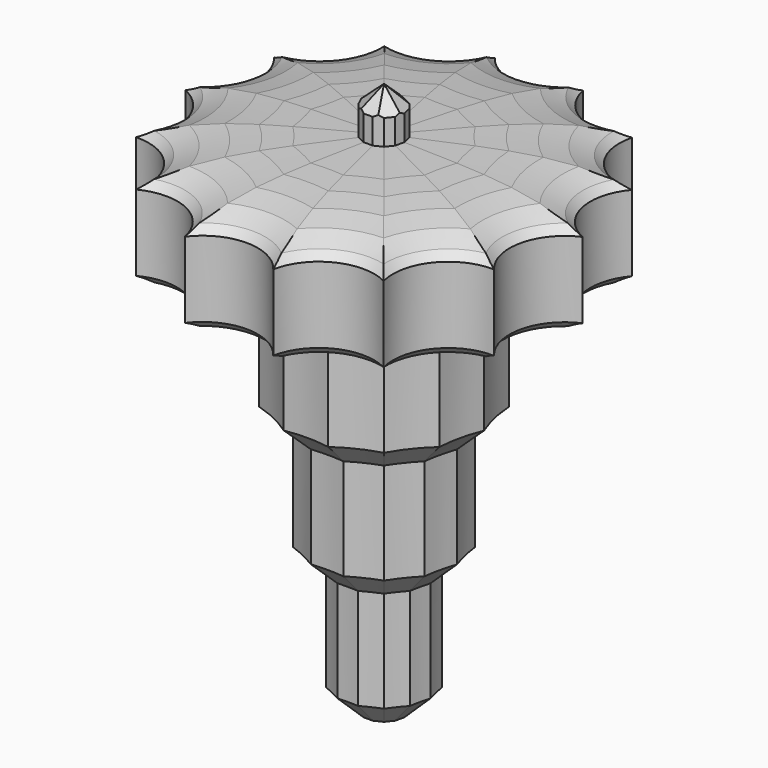
from build123d import *

# Parameters (mm, degrees)
F1_DEPTH      = 25
F2_T2_ANGLE   = 240.9081549798
F2_T4_ANGLE   = 240.9081549798
F2_T6_ANGLE   = 240.9081549797
F2_T8_ANGLE   = 240.9081549798
F2_T10_ANGLE  = 240.9081549798
F2_T12_ANGLE  = 240.9081549798
F2_T14_ANGLE  = 240.9081549798
F2_T16_ANGLE  = 240.9081549798
F2_T18_ANGLE  = 240.9081549798
F2_T20_ANGLE  = 240.9081549798
F2_T22_ANGLE  = 240.9081549798
F2_T24_ANGLE  = 240.9081549797
F2_T26_ANGLE  = 240.9081549798
F2_T28_ANGLE  = 240.9081549798
F3_SIZE       = 5
F4_SIZE       = 5
F5_SIZE       = 5
F6_T2_ANGLE   = 60.0762821523
F6_T4_ANGLE   = 60.0762821523
F6_T6_ANGLE   = 60.0762821523
F6_T8_ANGLE   = 60.0762821523
F6_T10_ANGLE  = 60.0762821523
F6_T12_ANGLE  = 60.0762821523
F6_T14_ANGLE  = 60.0762821523
F6_T16_ANGLE  = 60.0762821523
F6_T18_ANGLE  = 60.0762821523
F6_T20_ANGLE  = 60.0762821523
F6_T22_ANGLE  = 60.0762821523
F6_T24_ANGLE  = 60.0762821523
F6_T26_ANGLE  = 60.0762821523
F6_T28_ANGLE  = 60.0762821523
F7_T2_ANGLE   = 47.9835286681
F7_T4_ANGLE   = 47.9835286681
F7_T6_ANGLE   = 47.9835286681
F7_T8_ANGLE   = 47.9835286681
F7_T10_ANGLE  = 47.9835286681
F7_T12_ANGLE  = 47.9835286681
F7_T14_ANGLE  = 47.9835286681
F7_T16_ANGLE  = 47.9835286681
F7_T18_ANGLE  = 47.9835286681
F7_T20_ANGLE  = 47.9835286681
F7_T22_ANGLE  = 47.9835286681
F7_T24_ANGLE  = 47.9835286681
F7_T26_ANGLE  = 47.9835286681
F7_T28_ANGLE  = 47.9835286681
F8_T2_ANGLE   = 240.9081549798
F8_T4_ANGLE   = 240.9081549798
F8_T6_ANGLE   = 240.9081549798
F8_T8_ANGLE   = 240.9081549798
F8_T10_ANGLE  = 240.9081549798
F8_T12_ANGLE  = 240.9081549798
F8_T14_ANGLE  = 240.9081549797
F8_T16_ANGLE  = 240.9081549798
F8_T18_ANGLE  = 240.9081549797
F8_T20_ANGLE  = 240.9081549798
F8_T22_ANGLE  = 240.9081549798
F8_T24_ANGLE  = 240.9081549798
F8_T26_ANGLE  = 240.9081549798
F8_T28_ANGLE  = 240.9081549798
F9_SIZE       = 5
F10_SIZE      = 5
F11_DEPTH     = 25
F12_DEPTH     = 10
F13_T2_ANGLE  = 76.3607936653
F13_T4_ANGLE  = 76.3607936653
F13_T6_ANGLE  = 76.3607936653
F13_T8_ANGLE  = 76.3607936653
F13_T10_ANGLE = 76.3607936653
F13_T12_ANGLE = 76.3607936653
F13_T14_ANGLE = 76.3607936653
F13_T16_ANGLE = 76.3607936653
F13_T18_ANGLE = 76.3607936653
F13_T20_ANGLE = 76.3607936653
F13_T22_ANGLE = 76.3607936653
F13_T24_ANGLE = 76.3607936653
F13_T26_ANGLE = 76.3607936653
F13_T28_ANGLE = 76.3607936653
F13_T30_ANGLE = 38.4969644014
F13_T32_ANGLE = 38.4969644014
F13_T34_ANGLE = 38.4969644014
F13_T36_ANGLE = 38.4969644014
F13_T38_ANGLE = 38.4969644015
F13_T40_ANGLE = 38.4969644015
F13_T42_ANGLE = 38.4969644015
F15_DEPTH     = 25
F16_SIZE      = 5
F17_DEPTH     = 25
F18_SIZE      = 5


# Not quite as in the source:
# - a fillet or chamfer that OpenCascade refuses, or shapes differently, is made with other operations: its cross-section is extruded or revolved along the edge and cut away or added
# - two fillets or chamfers of one size are made in one step


with BuildPart() as f1:
    # F0 (on Top) → F1 (new body)
    with BuildSketch(Plane.XY):
        with BuildLine():
            ThreePointArc((24.463741661, 30.6765617538), (14.7080431141, 30.541566228), (8.731008312, 38.2530468191))
            ThreePointArc((8.731008312, 38.2530468191), (0, 33.8985810899), (-8.731008312, 38.2530468191))
            ThreePointArc((-8.731008312, 38.2530468191), (-14.7080431141, 30.541566228), (-24.463741661, 30.6765617538))
            ThreePointArc((-24.463741661, 30.6765617538), (-24.2050150864, 29.3243775762), (-24.1183144167, 27.9503963229))
            ThreePointArc((-24.1183144167, 27.9503963229), (-27.4274265196, 20.1152547902), (-35.351130946, 17.0242074097))
            ThreePointArc((-35.351130946, 17.0242074097), (-33.4389393825, 13.7278579439), (-32.7746255912, 9.9753809536))
            ThreePointArc((-32.7746255912, 9.9753809536), (-34.53133563, 4.0325730915), (-39.236795194, 0))
            ThreePointArc((-39.236795194, 0), (-34.53133563, -4.0325730915), (-32.7746255912, -9.9753809536))
            ThreePointArc((-32.7746255912, -9.9753809536), (-33.4389393825, -13.7278579439), (-35.351130946, -17.0242074097))
            ThreePointArc((-35.351130946, -17.0242074097), (-27.4274265195, -20.1152547902), (-24.1183144167, -27.9503963229))
            ThreePointArc((-24.1183144167, -27.9503963229), (-24.2050150864, -29.3243775762), (-24.463741661, -30.6765617538))
            ThreePointArc((-24.463741661, -30.6765617538), (-14.7080431141, -30.541566228), (-8.731008312, -38.2530468191))
            ThreePointArc((-8.731008312, -38.2530468191), (0, -33.8985810899), (8.731008312, -38.2530468191))
            ThreePointArc((8.731008312, -38.2530468191), (14.7080431141, -30.541566228), (24.463741661, -30.6765617538))
            ThreePointArc((24.463741661, -30.6765617538), (26.5029779071, -21.135419607), (35.351130946, -17.0242074097))
            ThreePointArc((35.351130946, -17.0242074097), (33.0486728879, -7.5431439239), (39.236795194, 0))
            ThreePointArc((39.236795194, 0), (33.0486728879, 7.5431439239), (35.351130946, 17.0242074097))
            ThreePointArc((35.351130946, 17.0242074097), (26.5029779071, 21.135419607), (24.463741661, 30.6765617538))
        make_face()
    extrude(amount=F1_DEPTH)

    # F2: chamfer of 5 on 14 edges, made by hand

    # F2_s1 → F2_t2 (revolve, cut)
    with BuildSketch(Plane(origin=(-13.8327660938, 36.0835914665, 0), x_dir=(0, 0, 1), z_dir=(-0.357952317, 0.9337398668, 0))):
        Polygon((25, -38.6518225177), (20, -33.6518225177), (25, -33.6518225177), align=None)
    revolve(axis=Axis((-35.0486884109, 27.9503963229, 25), (0, 0, 1)), revolution_arc=F2_T2_ANGLE, mode=Mode.SUBTRACT)

    # F2_s3 → F2_t4 (revolve, cut)
    with BuildSketch(Plane(origin=(-32.100820462, 21.5153042411, 0), x_dir=(0, 0, 1), z_dir=(-0.8306771749, 0.5567543723, 0))):
        Polygon((25, 38.6518225177), (20, 33.6518225177), (25, 33.6518225177), align=None)
    revolve(axis=Axis((-19.4505546526, 40.3894929114, 25), (0, 0, -1)), revolution_arc=F2_T4_ANGLE, mode=Mode.SUBTRACT)

    # F2_s5 → F2_t6 (revolve, cut)
    with BuildSketch(Plane(origin=(-19.586699218, 33.3126433155, 0), x_dir=(0, 0, 1), z_dir=(-0.5068476051, 0.8620356751, 0))):
        Polygon((25, 38.6518225177), (20, 33.6518225177), (25, 33.6518225177), align=None)
    revolve(axis=Axis((0, 44.8289550841, 25), (0, 0, -1)), revolution_arc=F2_T6_ANGLE, mode=Mode.SUBTRACT)

    # F2_s7 → F2_t8 (revolve, cut)
    with BuildSketch(Plane(origin=(-3.1931919788, 38.5120048285, 0), x_dir=(0, 0, 1), z_dir=(-0.082630651, 0.9965802404, 0))):
        Polygon((25, 38.6518225177), (20, 33.6518225177), (25, 33.6518225177), align=None)
    revolve(axis=Axis((19.4505546526, 40.3894929114, 25), (0, 0, -1)), revolution_arc=F2_T8_ANGLE, mode=Mode.SUBTRACT)

    # F2_s9 → F2_t10 (revolve, cut)
    with BuildSketch(Plane(origin=(13.8327660938, 36.0835914665, 0), x_dir=(0, 0, 1), z_dir=(0.357952317, 0.9337398668, 0))):
        Polygon((25, 38.6518225177), (20, 33.6518225177), (25, 33.6518225177), align=None)
    revolve(axis=Axis((35.0486884109, 27.9503963229, 25), (0, 0, -1)), revolution_arc=F2_T10_ANGLE, mode=Mode.SUBTRACT)

    # F2_s11 → F2_t12 (revolve, cut)
    with BuildSketch(Plane(origin=(28.1189751937, 26.5083802783, 0), x_dir=(0, 0, 1), z_dir=(0.7276384385, 0.685960861, 0))):
        Polygon((25, 38.6518225177), (20, 33.6518225177), (25, 33.6518225177), align=None)
    revolve(axis=Axis((43.7049995854, 9.9753809536, 25), (0, 0, -1)), revolution_arc=F2_T12_ANGLE, mode=Mode.SUBTRACT)

    # F2_s13 → F2_t14 (revolve, cut)
    with BuildSketch(Plane(origin=(36.8358764, 11.682859272, 0), x_dir=(0, 0, 1), z_dir=(0.9532068434, 0.3023188939, 0))):
        Polygon((25, 38.6518225177), (20, 33.6518225177), (25, 33.6518225177), align=None)
    revolve(axis=Axis((43.7049995854, -9.9753809536, 25), (0, 0, -1)), revolution_arc=F2_T14_ANGLE, mode=Mode.SUBTRACT)

    # F2_s15 → F2_t16 (revolve, cut)
    with BuildSketch(Plane(origin=(38.2569805228, -5.4565952939, 0), x_dir=(0, 0, 1), z_dir=(0.9899809427, -0.1412010378, 0))):
        Polygon((20, 33.6518225177), (25, 38.6518225177), (25, 33.6518225177), align=None)
    revolve(axis=Axis((35.0486884109, -27.9503963229, 25), (0, 0, -1)), revolution_arc=F2_T16_ANGLE, mode=Mode.SUBTRACT)

    # F2_s17 → F2_t18 (revolve, cut)
    with BuildSketch(Plane(origin=(32.100820462, -21.5153042411, 0), x_dir=(0, 0, 1), z_dir=(0.8306771749, -0.5567543723, 0))):
        Polygon((25, 38.6518225177), (20, 33.6518225177), (25, 33.6518225177), align=None)
    revolve(axis=Axis((19.4505546526, -40.3894929114, 25), (0, 0, -1)), revolution_arc=F2_T18_ANGLE, mode=Mode.SUBTRACT)

    # F2_s19 → F2_t20 (revolve, cut)
    with BuildSketch(Plane(origin=(19.586699218, -33.3126433155, 0), x_dir=(0, 0, 1), z_dir=(0.5068476051, -0.8620356751, 0))):
        Polygon((25, 38.6518225177), (20, 33.6518225177), (25, 33.6518225177), align=None)
    revolve(axis=Axis((0, -44.8289550841, 25), (0, 0, -1)), revolution_arc=F2_T20_ANGLE, mode=Mode.SUBTRACT)

    # F2_s21 → F2_t22 (revolve, cut)
    with BuildSketch(Plane(origin=(3.1931919788, -38.5120048285, 0), x_dir=(0, 0, 1), z_dir=(0.082630651, -0.9965802404, 0))):
        Polygon((25, 38.6518225177), (20, 33.6518225177), (25, 33.6518225177), align=None)
    revolve(axis=Axis((-19.4505546526, -40.3894929114, 25), (0, 0, -1)), revolution_arc=F2_T22_ANGLE, mode=Mode.SUBTRACT)

    # F2_s23 → F2_t24 (revolve, cut)
    with BuildSketch(Plane(origin=(-38.2569805228, -5.4565952939, 0), x_dir=(0, 0, 1), z_dir=(-0.9899809427, -0.1412010378, 0))):
        Polygon((25, -38.6518225177), (20, -33.6518225177), (25, -33.6518225177), align=None)
    revolve(axis=Axis((-35.0486884109, -27.9503963229, 25), (0, 0, 1)), revolution_arc=F2_T24_ANGLE, mode=Mode.SUBTRACT)

    # F2_s25 → F2_t26 (revolve, cut)
    with BuildSketch(Plane(origin=(-36.8358764, 11.682859272, 0), x_dir=(0, 0, 1), z_dir=(-0.9532068434, 0.3023188939, 0))):
        Polygon((25, -38.6518225177), (20, -33.6518225177), (25, -33.6518225177), align=None)
    revolve(axis=Axis((-43.7049995854, -9.9753809536, 25), (0, 0, 1)), revolution_arc=F2_T26_ANGLE, mode=Mode.SUBTRACT)

    # F2_s27 → F2_t28 (revolve, cut)
    with BuildSketch(Plane(origin=(-28.1189751937, 26.5083802783, 0), x_dir=(0, 0, 1), z_dir=(-0.7276384385, 0.685960861, 0))):
        Polygon((25, -38.6518225177), (20, -33.6518225177), (25, -33.6518225177), align=None)
    revolve(axis=Axis((-43.7049995854, 9.9753809536, 25), (0, 0, 1)), revolution_arc=F2_T28_ANGLE, mode=Mode.SUBTRACT)

    # F3
    f3_edges = [f1.edges().sort_by_distance(p)[0] for p in [
        (-22.59382, 18.017971, 25),
        (-12.538624, 26.036722, 25),
        (0, 28.898581, 25),
        (12.538624, 26.036722, 25),
        (22.59382, 18.017971, 25),
        (28.174033, 6.430539, 25),
        (28.174033, -6.430539, 25),
        (22.59382, -18.017971, 25),
        (12.538624, -26.036722, 25),
        (0, -28.898581, 25),
        (-12.538624, -26.036722, 25),
        (-22.59382, -18.017971, 25),
        (-28.174033, -6.430539, 25),
        (-28.174033, 6.430539, 25),
    ]]
    chamfer(f3_edges, length=F3_SIZE)

    # F4
    f4_edges = [f1.edges().sort_by_distance(p)[0] for p in [
        (-18.684663, 14.900522, 25),
        (-10.369206, 21.531878, 25),
        (0, 23.898581, 25),
        (10.369206, 21.531878, 25),
        (18.684663, 14.900522, 25),
        (23.299394, 5.317935, 25),
        (23.299394, -5.317935, 25),
        (18.684663, -14.900522, 25),
        (10.369206, -21.531878, 25),
        (0, -23.898581, 25),
        (-10.369206, -21.531878, 25),
        (-18.684663, -14.900522, 25),
        (-23.299394, -5.317935, 25),
        (-23.299394, 5.317935, 25),
    ]]
    chamfer(f4_edges, length=F4_SIZE)

    # F5
    f5_edges = [f1.edges().sort_by_distance(p)[0] for p in [
        (-14.775506, 11.783073, 25),
        (-18.424754, 4.20533, 25),
        (-18.424754, -4.20533, 25),
        (-14.775506, -11.783073, 25),
        (-8.199787, -17.027033, 25),
        (0, -18.898581, 25),
        (8.199787, -17.027033, 25),
        (14.775506, -11.783073, 25),
        (-8.199787, 17.027033, 25),
        (0, 18.898581, 25),
        (8.199787, 17.027033, 25),
        (14.775506, 11.783073, 25),
        (18.424754, 4.20533, 25),
        (18.424754, -4.20533, 25),
    ]]
    chamfer(f5_edges, length=F5_SIZE)

    # F6: chamfer of 5 on 14 edges, made by hand

    # F6_s1 → F6_t2 (revolve, cut)
    with BuildSketch(Plane(origin=(-20.8945545214, -8.184460814, 0), x_dir=(0, 0, 1), z_dir=(-0.9311167453, -0.3647212726, 0))):
        Polygon((25, 2.8777102985), (24.5099142984, 12.8536339319), (25, 7.8777102985), align=None)
    revolve(axis=Axis((-35.0486884109, 27.9503963229, 25), (0, 0, 1)), revolution_arc=F6_T2_ANGLE, mode=Mode.SUBTRACT)

    # F6_s3 → F6_t4 (revolve, cut)
    with BuildSketch(Plane(origin=(-15.2742386719, -16.4397518369, 0), x_dir=(0, 0, 1), z_dir=(-0.6806605704, -0.732598927, 0))):
        Polygon((25, 2.8777102985), (24.5099142984, 12.8536339319), (25, 7.8777102985), align=None)
    revolve(axis=Axis((-43.7049995854, 9.9753809536, 25), (0, 0, 1)), revolution_arc=F6_T4_ANGLE, mode=Mode.SUBTRACT)

    # F6_s5 → F6_t6 (revolve, cut)
    with BuildSketch(Plane(origin=(12.6287350804, 18.5494705513, 0), x_dir=(0, 0, 1), z_dir=(0.5627699166, 0.8266135863, 0))):
        Polygon((25, -2.8777102985), (24.5099142984, -12.8536339319), (25, -7.8777102985), align=None)
    revolve(axis=Axis((-19.4505546526, 40.3894929114, 25), (0, 0, -1)), revolution_arc=F6_T6_ANGLE, mode=Mode.SUBTRACT)

    # F6_s7 → F6_t8 (revolve, cut)
    with BuildSketch(Plane(origin=(-6.6286725271, -21.4389483882, 0), x_dir=(0, 0, 1), z_dir=(-0.2953912218, -0.9553763793, 0))):
        Polygon((25, 2.8777102985), (24.5099142984, 12.8536339319), (25, 7.8777102985), align=None)
    revolve(axis=Axis((-43.7049995854, -9.9753809536, 25), (0, 0, 1)), revolution_arc=F6_T8_ANGLE, mode=Mode.SUBTRACT)

    # F6_s9 → F6_t10 (revolve, cut)
    with BuildSketch(Plane(origin=(19.4264107899, 11.2330926858, 0), x_dir=(0, 0, 1), z_dir=(0.8656923682, 0.5005763913, 0))):
        Polygon((25, -2.8777102985), (24.5099142984, -12.8536339318), (25, -7.8777102985), align=None)
    revolve(axis=Axis((0, 44.8289550841, 25), (0, 0, -1)), revolution_arc=F6_T10_ANGLE, mode=Mode.SUBTRACT)

    # F6_s11 → F6_t12 (revolve, cut)
    with BuildSketch(Plane(origin=(3.329783507, -22.1918982798, 0), x_dir=(0, 0, 1), z_dir=(0.148383981, -0.9889298227, 0))):
        Polygon((25, 2.8777102985), (24.5099142984, 12.8536339318), (25, 7.8777102985), align=None)
    revolve(axis=Axis((-35.0486884109, -27.9503963229, 25), (0, 0, 1)), revolution_arc=F6_T12_ANGLE, mode=Mode.SUBTRACT)

    # F6_s13 → F6_t14 (revolve, cut)
    with BuildSketch(Plane(origin=(22.3764475931, 1.691863049, 0), x_dir=(0, 0, 1), z_dir=(0.9971538294, 0.0753939029, 0))):
        Polygon((25, -2.8777102985), (24.5099142984, -12.8536339319), (25, -7.8777102985), align=None)
    revolve(axis=Axis((19.4505546526, 40.3894929114, 25), (0, 0, -1)), revolution_arc=F6_T14_ANGLE, mode=Mode.SUBTRACT)

    # F6_s15 → F6_t16 (revolve, cut)
    with BuildSketch(Plane(origin=(-22.3764475931, -1.691863049, 0), x_dir=(0, 0, 1), z_dir=(-0.9971538294, -0.0753939029, 0))):
        Polygon((25, -2.8777102985), (24.5099142984, -12.8536339319), (25, -7.8777102985), align=None)
    revolve(axis=Axis((-19.4505546526, -40.3894929114, 25), (0, 0, -1)), revolution_arc=F6_T16_ANGLE, mode=Mode.SUBTRACT)

    # F6_s17 → F6_t18 (revolve, cut)
    with BuildSketch(Plane(origin=(20.8945545214, -8.184460814, 0), x_dir=(0, 0, 1), z_dir=(0.9311167453, -0.3647212726, 0))):
        Polygon((25, -2.8777102985), (24.5099142984, -12.8536339319), (25, -7.8777102985), align=None)
    revolve(axis=Axis((35.0486884109, 27.9503963229, 25), (0, 0, -1)), revolution_arc=F6_T18_ANGLE, mode=Mode.SUBTRACT)

    # F6_s19 → F6_t20 (revolve, cut)
    with BuildSketch(Plane(origin=(-19.4264107899, -11.2330926858, 0), x_dir=(0, 0, 1), z_dir=(-0.8656923682, -0.5005763913, 0))):
        Polygon((25, -2.8777102985), (24.5099142984, -12.8536339318), (25, -7.8777102985), align=None)
    revolve(axis=Axis((0, -44.8289550841, 25), (0, 0, -1)), revolution_arc=F6_T20_ANGLE, mode=Mode.SUBTRACT)

    # F6_s21 → F6_t22 (revolve, cut)
    with BuildSketch(Plane(origin=(15.2742386718, -16.4397518369, 0), x_dir=(0, 0, 1), z_dir=(0.6806605704, -0.732598927, 0))):
        Polygon((25, -2.8777102985), (24.5099142984, -12.8536339319), (25, -7.8777102985), align=None)
    revolve(axis=Axis((43.7049995854, 9.9753809536, 25), (0, 0, -1)), revolution_arc=F6_T22_ANGLE, mode=Mode.SUBTRACT)

    # F6_s23 → F6_t24 (revolve, cut)
    with BuildSketch(Plane(origin=(-12.6287350804, -18.5494705513, 0), x_dir=(0, 0, 1), z_dir=(-0.5627699166, -0.8266135863, 0))):
        Polygon((24.5099142984, -12.8536339319), (25, -2.8777102985), (25, -7.8777102985), align=None)
    revolve(axis=Axis((19.4505546526, -40.3894929114, 25), (0, 0, -1)), revolution_arc=F6_T24_ANGLE, mode=Mode.SUBTRACT)

    # F6_s25 → F6_t26 (revolve, cut)
    with BuildSketch(Plane(origin=(6.6286725271, -21.4389483882, 0), x_dir=(0, 0, 1), z_dir=(0.2953912218, -0.9553763793, 0))):
        Polygon((25, -2.8777102985), (24.5099142984, -12.8536339318), (25, -7.8777102985), align=None)
    revolve(axis=Axis((43.7049995854, -9.9753809536, 25), (0, 0, -1)), revolution_arc=F6_T26_ANGLE, mode=Mode.SUBTRACT)

    # F6_s27 → F6_t28 (revolve, cut)
    with BuildSketch(Plane(origin=(-3.329783507, -22.1918982798, 0), x_dir=(0, 0, 1), z_dir=(-0.148383981, -0.9889298227, 0))):
        Polygon((24.5099142984, -12.8536339319), (25, -2.8777102985), (25, -7.8777102985), align=None)
    revolve(axis=Axis((35.0486884109, -27.9503963229, 25), (0, 0, -1)), revolution_arc=F6_T28_ANGLE, mode=Mode.SUBTRACT)

    # F7: chamfer of 5 on 14 edges, made by hand

    # F7_s1 → F7_t2 (revolve, cut)
    with BuildSketch(Plane(origin=(-16.1774332378, -8.3987740904, 0), x_dir=(0, 0, 1), z_dir=(-0.8875195673, -0.4607700268, 0))):
        Polygon((25, 0.0255347559), (24.7546616284, 10.019512037), (25, 5.0255347559), align=None)
    revolve(axis=Axis((-35.0486884109, 27.9503963229, 25), (0, 0, 1)), revolution_arc=F7_T2_ANGLE, mode=Mode.SUBTRACT)

    # F7_s3 → F7_t4 (revolve, cut)
    with BuildSketch(Plane(origin=(11.7880168419, 13.9029281563, 0), x_dir=(0, 0, 1), z_dir=(0.6467092433, 0.7627366221, 0))):
        Polygon((25, -0.0255347559), (24.7546616284, -10.019512037), (25, -5.0255347559), align=None)
    revolve(axis=Axis((-19.4505546526, 40.3894929114, 25), (0, 0, -1)), revolution_arc=F7_T4_ANGLE, mode=Mode.SUBTRACT)

    # F7_s5 → F7_t6 (revolve, cut)
    with BuildSketch(Plane(origin=(16.652890642, 7.4114766173, 0), x_dir=(0, 0, 1), z_dir=(0.9136039123, 0.4066053263, 0))):
        Polygon((25, -0.0255347559), (24.7546616284, -10.019512037), (25, -5.0255347559), align=None)
    revolve(axis=Axis((0, 44.8289550841, 25), (0, 0, -1)), revolution_arc=F7_T6_ANGLE, mode=Mode.SUBTRACT)

    # F7_s7 → F7_t8 (revolve, cut)
    with BuildSketch(Plane(origin=(18.2194552162, -0.5479087615, 0), x_dir=(0, 0, 1), z_dir=(0.9995481219, -0.030059141, 0))):
        Polygon((25, -0.0255347559), (24.7546616284, -10.019512037), (25, -5.0255347559), align=None)
    revolve(axis=Axis((19.4505546526, 40.3894929114, 25), (0, 0, -1)), revolution_arc=F7_T8_ANGLE, mode=Mode.SUBTRACT)

    # F7_s9 → F7_t10 (revolve, cut)
    with BuildSketch(Plane(origin=(16.1774332378, -8.3987740904, 0), x_dir=(0, 0, 1), z_dir=(0.8875195673, -0.4607700268, 0))):
        Polygon((25, -0.0255347559), (24.7546616284, -10.019512037), (25, -5.0255347559), align=None)
    revolve(axis=Axis((35.0486884109, 27.9503963229, 25), (0, 0, -1)), revolution_arc=F7_T10_ANGLE, mode=Mode.SUBTRACT)

    # F7_s11 → F7_t12 (revolve, cut)
    with BuildSketch(Plane(origin=(10.9312722034, -14.5861592065, 0), x_dir=(0, 0, 1), z_dir=(0.5997068777, -0.8002197578, 0))):
        Polygon((25, -0.0255347559), (24.7546616284, -10.019512037), (25, -5.0255347559), align=None)
    revolve(axis=Axis((43.7049995854, 9.9753809536, 25), (0, 0, -1)), revolution_arc=F7_T12_ANGLE, mode=Mode.SUBTRACT)

    # F7_s13 → F7_t14 (revolve, cut)
    with BuildSketch(Plane(origin=(3.520038646, -17.8845766043, 0), x_dir=(0, 0, 1), z_dir=(0.193114886, -0.9811761518, 0))):
        Polygon((25, -0.0255347559), (24.7546616284, -10.019512037), (25, -5.0255347559), align=None)
    revolve(axis=Axis((43.7049995854, -9.9753809536, 25), (0, 0, -1)), revolution_arc=F7_T14_ANGLE, mode=Mode.SUBTRACT)

    # F7_s15 → F7_t16 (revolve, cut)
    with BuildSketch(Plane(origin=(-4.5883817358, -17.6407342656, 0), x_dir=(0, 0, 1), z_dir=(-0.2517258772, -0.9677985755, 0))):
        Polygon((24.7546616284, -10.019512037), (25, -0.0255347559), (25, -5.0255347559), align=None)
    revolve(axis=Axis((35.0486884109, -27.9503963229, 25), (0, 0, -1)), revolution_arc=F7_T16_ANGLE, mode=Mode.SUBTRACT)

    # F7_s17 → F7_t18 (revolve, cut)
    with BuildSketch(Plane(origin=(-11.7880168419, -13.9029281563, 0), x_dir=(0, 0, 1), z_dir=(-0.6467092433, -0.7627366221, 0))):
        Polygon((24.7546616284, -10.019512037), (25, -0.0255347559), (25, -5.0255347559), align=None)
    revolve(axis=Axis((19.4505546526, -40.3894929114, 25), (0, 0, -1)), revolution_arc=F7_T18_ANGLE, mode=Mode.SUBTRACT)

    # F7_s19 → F7_t20 (revolve, cut)
    with BuildSketch(Plane(origin=(-16.652890642, -7.4114766173, 0), x_dir=(0, 0, 1), z_dir=(-0.9136039123, -0.4066053263, 0))):
        Polygon((25, -0.0255347559), (24.7546616284, -10.019512037), (25, -5.0255347559), align=None)
    revolve(axis=Axis((0, -44.8289550841, 25), (0, 0, -1)), revolution_arc=F7_T20_ANGLE, mode=Mode.SUBTRACT)

    # F7_s21 → F7_t22 (revolve, cut)
    with BuildSketch(Plane(origin=(-18.2194552162, 0.5479087615, 0), x_dir=(0, 0, 1), z_dir=(-0.9995481219, 0.030059141, 0))):
        Polygon((25, -0.0255347559), (24.7546616284, -10.019512037), (25, -5.0255347559), align=None)
    revolve(axis=Axis((-19.4505546526, -40.3894929114, 25), (0, 0, -1)), revolution_arc=F7_T22_ANGLE, mode=Mode.SUBTRACT)

    # F7_s23 → F7_t24 (revolve, cut)
    with BuildSketch(Plane(origin=(4.5883817358, -17.6407342656, 0), x_dir=(0, 0, 1), z_dir=(0.2517258772, -0.9677985755, 0))):
        Polygon((25, 0.0255347559), (24.7546616284, 10.019512037), (25, 5.0255347559), align=None)
    revolve(axis=Axis((-35.0486884109, -27.9503963229, 25), (0, 0, 1)), revolution_arc=F7_T24_ANGLE, mode=Mode.SUBTRACT)

    # F7_s25 → F7_t26 (revolve, cut)
    with BuildSketch(Plane(origin=(-3.520038646, -17.8845766043, 0), x_dir=(0, 0, 1), z_dir=(-0.193114886, -0.9811761518, 0))):
        Polygon((25, 0.0255347559), (24.7546616284, 10.019512037), (25, 5.0255347559), align=None)
    revolve(axis=Axis((-43.7049995854, -9.9753809536, 25), (0, 0, 1)), revolution_arc=F7_T26_ANGLE, mode=Mode.SUBTRACT)

    # F7_s27 → F7_t28 (revolve, cut)
    with BuildSketch(Plane(origin=(-10.9312722034, -14.5861592065, 0), x_dir=(0, 0, 1), z_dir=(-0.5997068777, -0.8002197578, 0))):
        Polygon((25, 0.0255347559), (24.7546616284, 10.019512037), (25, 5.0255347559), align=None)
    revolve(axis=Axis((-43.7049995854, 9.9753809536, 25), (0, 0, 1)), revolution_arc=F7_T28_ANGLE, mode=Mode.SUBTRACT)

    # F8: chamfer of 5 on 14 edges, made by hand

    # F8_s1 → F8_t2 (revolve, cut)
    with BuildSketch(Plane(origin=(-28.1189751937, -26.5083802783, 0), x_dir=(0, 0, 1), z_dir=(-0.7276384385, -0.685960861, 0))):
        Polygon((0, 38.6518225177), (5, 33.6518225177), (0, 33.6518225177), align=None)
    revolve(axis=Axis((-43.7049995854, -9.9753809536, 0), (0, 0, -1)), revolution_arc=F8_T2_ANGLE, mode=Mode.SUBTRACT)

    # F8_s3 → F8_t4 (revolve, cut)
    with BuildSketch(Plane(origin=(38.2569805228, -5.4565952939, 0), x_dir=(0, 0, 1), z_dir=(0.9899809427, -0.1412010378, 0))):
        Polygon((5, 33.6518225177), (0, 38.6518225177), (0, 33.6518225177), align=None)
    revolve(axis=Axis((35.0486884109, -27.9503963229, 0), (0, 0, -1)), revolution_arc=F8_T4_ANGLE, mode=Mode.SUBTRACT)

    # F8_s5 → F8_t6 (revolve, cut)
    with BuildSketch(Plane(origin=(36.8358764, 11.682859272, 0), x_dir=(0, 0, 1), z_dir=(0.9532068434, 0.3023188939, 0))):
        Polygon((0, 38.6518225177), (5, 33.6518225177), (0, 33.6518225177), align=None)
    revolve(axis=Axis((43.7049995854, -9.9753809536, 0), (0, 0, -1)), revolution_arc=F8_T6_ANGLE, mode=Mode.SUBTRACT)

    # F8_s7 → F8_t8 (revolve, cut)
    with BuildSketch(Plane(origin=(28.1189751937, 26.5083802783, 0), x_dir=(0, 0, 1), z_dir=(0.7276384385, 0.685960861, 0))):
        Polygon((0, 38.6518225177), (5, 33.6518225177), (0, 33.6518225177), align=None)
    revolve(axis=Axis((43.7049995854, 9.9753809536, 0), (0, 0, -1)), revolution_arc=F8_T8_ANGLE, mode=Mode.SUBTRACT)

    # F8_s9 → F8_t10 (revolve, cut)
    with BuildSketch(Plane(origin=(13.8327660938, 36.0835914665, 0), x_dir=(0, 0, 1), z_dir=(0.357952317, 0.9337398668, 0))):
        Polygon((0, 38.6518225177), (5, 33.6518225177), (0, 33.6518225177), align=None)
    revolve(axis=Axis((35.0486884109, 27.9503963229, 0), (0, 0, -1)), revolution_arc=F8_T10_ANGLE, mode=Mode.SUBTRACT)

    # F8_s11 → F8_t12 (revolve, cut)
    with BuildSketch(Plane(origin=(-3.1931919788, 38.5120048285, 0), x_dir=(0, 0, 1), z_dir=(-0.082630651, 0.9965802404, 0))):
        Polygon((0, 38.6518225177), (5, 33.6518225177), (0, 33.6518225177), align=None)
    revolve(axis=Axis((19.4505546526, 40.3894929114, 0), (0, 0, -1)), revolution_arc=F8_T12_ANGLE, mode=Mode.SUBTRACT)

    # F8_s13 → F8_t14 (revolve, cut)
    with BuildSketch(Plane(origin=(-19.586699218, 33.3126433155, 0), x_dir=(0, 0, 1), z_dir=(-0.5068476051, 0.8620356751, 0))):
        Polygon((0, 38.6518225177), (5, 33.6518225177), (0, 33.6518225177), align=None)
    revolve(axis=Axis((0, 44.8289550841, 0), (0, 0, -1)), revolution_arc=F8_T14_ANGLE, mode=Mode.SUBTRACT)

    # F8_s15 → F8_t16 (revolve, cut)
    with BuildSketch(Plane(origin=(-32.100820462, 21.5153042411, 0), x_dir=(0, 0, 1), z_dir=(-0.8306771749, 0.5567543723, 0))):
        Polygon((0, 38.6518225177), (5, 33.6518225177), (0, 33.6518225177), align=None)
    revolve(axis=Axis((-19.4505546526, 40.3894929114, 0), (0, 0, -1)), revolution_arc=F8_T16_ANGLE, mode=Mode.SUBTRACT)

    # F8_s17 → F8_t18 (revolve, cut)
    with BuildSketch(Plane(origin=(-38.2569805228, 5.4565952939, 0), x_dir=(0, 0, 1), z_dir=(-0.9899809427, 0.1412010378, 0))):
        Polygon((0, 38.6518225177), (5, 33.6518225177), (0, 33.6518225177), align=None)
    revolve(axis=Axis((-35.0486884109, 27.9503963229, 0), (0, 0, -1)), revolution_arc=F8_T18_ANGLE, mode=Mode.SUBTRACT)

    # F8_s19 → F8_t20 (revolve, cut)
    with BuildSketch(Plane(origin=(-36.8358764, -11.682859272, 0), x_dir=(0, 0, 1), z_dir=(-0.9532068434, -0.3023188939, 0))):
        Polygon((0, 38.6518225177), (5, 33.6518225177), (0, 33.6518225177), align=None)
    revolve(axis=Axis((-43.7049995854, 9.9753809536, 0), (0, 0, -1)), revolution_arc=F8_T20_ANGLE, mode=Mode.SUBTRACT)

    # F8_s21 → F8_t22 (revolve, cut)
    with BuildSketch(Plane(origin=(-13.8327660938, -36.0835914665, 0), x_dir=(0, 0, 1), z_dir=(-0.357952317, -0.9337398668, 0))):
        Polygon((0, 38.6518225177), (5, 33.6518225177), (0, 33.6518225177), align=None)
    revolve(axis=Axis((-35.0486884109, -27.9503963229, 0), (0, 0, -1)), revolution_arc=F8_T22_ANGLE, mode=Mode.SUBTRACT)

    # F8_s23 → F8_t24 (revolve, cut)
    with BuildSketch(Plane(origin=(3.1931919788, -38.5120048285, 0), x_dir=(0, 0, 1), z_dir=(0.082630651, -0.9965802404, 0))):
        Polygon((0, 38.6518225177), (5, 33.6518225177), (0, 33.6518225177), align=None)
    revolve(axis=Axis((-19.4505546526, -40.3894929114, 0), (0, 0, -1)), revolution_arc=F8_T24_ANGLE, mode=Mode.SUBTRACT)

    # F8_s25 → F8_t26 (revolve, cut)
    with BuildSketch(Plane(origin=(19.586699218, -33.3126433155, 0), x_dir=(0, 0, 1), z_dir=(0.5068476051, -0.8620356751, 0))):
        Polygon((0, 38.6518225177), (5, 33.6518225177), (0, 33.6518225177), align=None)
    revolve(axis=Axis((0, -44.8289550841, 0), (0, 0, -1)), revolution_arc=F8_T26_ANGLE, mode=Mode.SUBTRACT)

    # F8_s27 → F8_t28 (revolve, cut)
    with BuildSketch(Plane(origin=(32.100820462, -21.5153042411, 0), x_dir=(0, 0, 1), z_dir=(0.8306771749, -0.5567543723, 0))):
        Polygon((5, 33.6518225177), (0, 38.6518225177), (0, 33.6518225177), align=None)
    revolve(axis=Axis((19.4505546526, -40.3894929114, 0), (0, 0, -1)), revolution_arc=F8_T28_ANGLE, mode=Mode.SUBTRACT)

    # F9
    f9_edges = [f1.edges().sort_by_distance(p)[0] for p in [
        (22.59382, -18.017971, 0),
        (12.538624, -26.036722, 0),
        (0, -28.898581, 0),
        (-12.538624, -26.036722, 0),
        (-22.59382, -18.017971, 0),
        (-28.174033, -6.430539, 0),
        (-28.174033, 6.430539, 0),
        (-22.59382, 18.017971, 0),
        (-12.538624, 26.036722, 0),
        (0, 28.898581, 0),
        (12.538624, 26.036722, 0),
        (22.59382, 18.017971, 0),
        (28.174033, 6.430539, 0),
        (28.174033, -6.430539, 0),
    ]]
    chamfer(f9_edges, length=F9_SIZE)

    # F10
    f10_edges = [f1.edges().sort_by_distance(p)[0] for p in [
        (18.684663, -14.900522, 0),
        (10.369206, -21.531878, 0),
        (23.299394, -5.317935, 0),
        (0, -23.898581, 0),
        (23.299394, 5.317935, 0),
        (-10.369206, -21.531878, 0),
        (18.684663, 14.900522, 0),
        (-18.684663, -14.900522, 0),
        (10.369206, 21.531878, 0),
        (-23.299394, -5.317935, 0),
        (0, 23.898581, 0),
        (-23.299394, 5.317935, 0),
        (-10.369206, 21.531878, 0),
        (-18.684663, 14.900522, 0),
    ]]
    chamfer(f10_edges, length=F10_SIZE)

    # F11 (add): a face of the model
    f11_faces = [f1.faces().sort_by_distance(p)[0] for p in [
        (0, 0, 0),
    ]]
    extrude(f11_faces, amount=F11_DEPTH)

    # F12 (add): a face of the model
    f12_faces = [f1.faces().sort_by_distance(p)[0] for p in [
        (0, 0, 25),
    ]]
    extrude(f12_faces, amount=F12_DEPTH)

    # F13: chamfer of 5 on 21 edges, made by hand

    # F13_s1 → F13_t2 (revolve, cut)
    with BuildSketch(Plane(origin=(-0.1891172344, -27.7099019188, 0), x_dir=(0, 0, 1), z_dir=(-0.0068247383, -0.9999767112, 0))):
        Polygon((-20, -9.3082523163), (-25, -4.3082523163), (-25, -9.3082523163), align=None)
    revolve(axis=Axis((35.0486884109, -27.9503963229, -25), (0, 0, -1)), revolution_arc=F13_T2_ANGLE, mode=Mode.SUBTRACT)

    # F13_s3 → F13_t4 (revolve, cut)
    with BuildSketch(Plane(origin=(-12.1932645957, -24.8837040687, 0), x_dir=(0, 0, 1), z_dir=(-0.4400225113, -0.8979867424, 0))):
        Polygon((-20, -9.3082523163), (-25, -4.3082523163), (-25, -9.3082523163), align=None)
    revolve(axis=Axis((19.4505546526, -40.3894929114, -25), (0, 0, -1)), revolution_arc=F13_T4_ANGLE, mode=Mode.SUBTRACT)

    # F13_s5 → F13_t6 (revolve, cut)
    with BuildSketch(Plane(origin=(11.8524871146, -25.0478138543, 0), x_dir=(0, 0, 1), z_dir=(0.4277247577, -0.9039090284, 0))):
        Polygon((-20, -9.3082523163), (-25, -4.3082523163), (-25, -9.3082523163), align=None)
    revolve(axis=Axis((43.7049995854, -9.9753809536, -25), (0, 0, -1)), revolution_arc=F13_T6_ANGLE, mode=Mode.SUBTRACT)

    # F13_s7 → F13_t8 (revolve, cut)
    with BuildSketch(Plane(origin=(-21.7823863632, -17.1289834492, 0), x_dir=(0, 0, 1), z_dir=(-0.7860684293, -0.6181394862, 0))):
        Polygon((-25, -4.3082523163), (-20, -9.3082523163), (-25, -9.3082523163), align=None)
    revolve(axis=Axis((0, -44.8289550841, -25), (0, 0, -1)), revolution_arc=F13_T8_ANGLE, mode=Mode.SUBTRACT)

    # F13_s9 → F13_t10 (revolve, cut)
    with BuildSketch(Plane(origin=(21.5465610293, -17.4246990646, 0), x_dir=(0, 0, 1), z_dir=(0.7775581198, -0.6288110768, 0))):
        Polygon((-25, -4.3082523163), (-20, -9.3082523163), (-25, -9.3082523163), align=None)
    revolve(axis=Axis((43.7049995854, 9.9753809536, -25), (0, 0, -1)), revolution_arc=F13_T10_ANGLE, mode=Mode.SUBTRACT)

    # F13_s11 → F13_t12 (revolve, cut)
    with BuildSketch(Plane(origin=(-27.0572393681, -5.9816575844, 0), x_dir=(0, 0, 1), z_dir=(-0.9764238544, -0.2158621238, 0))):
        Polygon((-25, -4.3082523163), (-20, -9.3082523163), (-25, -9.3082523163), align=None)
    revolve(axis=Axis((-19.4505546526, -40.3894929114, -25), (0, 0, -1)), revolution_arc=F13_T12_ANGLE, mode=Mode.SUBTRACT)

    # F13_s13 → F13_t14 (revolve, cut)
    with BuildSketch(Plane(origin=(26.9730742809, -6.3504089253, 0), x_dir=(0, 0, 1), z_dir=(0.9733865601, -0.2291693796, 0))):
        Polygon((-25, -4.3082523163), (-20, -9.3082523163), (-25, -9.3082523163), align=None)
    revolve(axis=Axis((35.0486884109, 27.9503963229, -25), (0, 0, -1)), revolution_arc=F13_T14_ANGLE, mode=Mode.SUBTRACT)

    # F13_s15 → F13_t16 (revolve, cut)
    with BuildSketch(Plane(origin=(-26.9730742809, 6.3504089253, 0), x_dir=(0, 0, 1), z_dir=(-0.9733865601, 0.2291693796, 0))):
        Polygon((-25, -4.3082523163), (-20, -9.3082523163), (-25, -9.3082523163), align=None)
    revolve(axis=Axis((-35.0486884109, -27.9503963229, -25), (0, 0, -1)), revolution_arc=F13_T16_ANGLE, mode=Mode.SUBTRACT)

    # F13_s17 → F13_t18 (revolve, cut)
    with BuildSketch(Plane(origin=(27.0572393681, 5.9816575844, 0), x_dir=(0, 0, 1), z_dir=(0.9764238544, 0.2158621238, 0))):
        Polygon((-25, -4.3082523163), (-20, -9.3082523163), (-25, -9.3082523163), align=None)
    revolve(axis=Axis((19.4505546526, 40.3894929114, -25), (0, 0, -1)), revolution_arc=F13_T18_ANGLE, mode=Mode.SUBTRACT)

    # F13_s19 → F13_t20 (revolve, cut)
    with BuildSketch(Plane(origin=(-21.5465610293, 17.4246990646, 0), x_dir=(0, 0, 1), z_dir=(-0.7775581198, 0.6288110768, 0))):
        Polygon((-25, -4.3082523163), (-20, -9.3082523163), (-25, -9.3082523163), align=None)
    revolve(axis=Axis((-43.7049995854, -9.9753809536, -25), (0, 0, -1)), revolution_arc=F13_T20_ANGLE, mode=Mode.SUBTRACT)

    # F13_s21 → F13_t22 (revolve, cut)
    with BuildSketch(Plane(origin=(21.7823863632, 17.1289834492, 0), x_dir=(0, 0, 1), z_dir=(0.7860684293, 0.6181394862, 0))):
        Polygon((-25, -4.3082523163), (-20, -9.3082523163), (-25, -9.3082523163), align=None)
    revolve(axis=Axis((0, 44.8289550841, -25), (0, 0, -1)), revolution_arc=F13_T22_ANGLE, mode=Mode.SUBTRACT)

    # F13_s23 → F13_t24 (revolve, cut)
    with BuildSketch(Plane(origin=(-11.8524871146, 25.0478138543, 0), x_dir=(0, 0, 1), z_dir=(-0.4277247577, 0.9039090284, 0))):
        Polygon((-25, -4.3082523163), (-20, -9.3082523163), (-25, -9.3082523163), align=None)
    revolve(axis=Axis((-43.7049995854, 9.9753809536, -25), (0, 0, -1)), revolution_arc=F13_T24_ANGLE, mode=Mode.SUBTRACT)

    # F13_s25 → F13_t26 (revolve, cut)
    with BuildSketch(Plane(origin=(12.1932645957, 24.8837040687, 0), x_dir=(0, 0, 1), z_dir=(0.4400225113, 0.8979867424, 0))):
        Polygon((-25, -4.3082523163), (-20, -9.3082523163), (-25, -9.3082523163), align=None)
    revolve(axis=Axis((-19.4505546526, 40.3894929114, -25), (0, 0, -1)), revolution_arc=F13_T26_ANGLE, mode=Mode.SUBTRACT)

    # F13_s27 → F13_t28 (revolve, cut)
    with BuildSketch(Plane(origin=(0.1891172344, 27.7099019188, 0), x_dir=(0, 0, 1), z_dir=(0.0068247383, 0.9999767112, 0))):
        Polygon((-25, -4.3082523163), (-20, -9.3082523163), (-25, -9.3082523163), align=None)
    revolve(axis=Axis((-35.0486884109, 27.9503963229, -25), (0, 0, -1)), revolution_arc=F13_T28_ANGLE, mode=Mode.SUBTRACT)

    # F13_s29 → F13_t30 (revolve, cut)
    with BuildSketch(Plane(origin=(-4.8901144067, -13.9460673073, 0), x_dir=(0, 0, 1), z_dir=(-0.3308923488, -0.9436685083, 0))):
        Polygon((30, -1.3925418042), (35, 3.6074581958), (35, -1.3925418042), align=None)
    revolve(axis=Axis((35.0486884109, -27.9503963229, 35), (0, 0, -1)), revolution_arc=F13_T30_ANGLE, mode=Mode.SUBTRACT)

    # F13_s31 → F13_t32 (revolve, cut)
    with BuildSketch(Plane(origin=(10.4568126702, 10.4432313501, 0), x_dir=(0, 0, 1), z_dir=(0.7075661257, 0.706647138, 0))):
        Polygon((35, 3.6074581958), (30, -1.3925418042), (35, -1.3925418042), align=None)
    revolve(axis=Axis((-19.4505546526, 40.3894929114, 35), (0, 0, -1)), revolution_arc=F13_T32_ANGLE, mode=Mode.SUBTRACT)

    # F13_s33 → F13_t34 (revolve, cut)
    with BuildSketch(Plane(origin=(14.684563108, -1.6642171066, 0), x_dir=(0, 0, 1), z_dir=(0.9936392431, -0.1126101889, 0))):
        Polygon((35, 3.6074581958), (30, -1.3925418042), (35, -1.3925418042), align=None)
    revolve(axis=Axis((19.4505546526, 40.3894929114, 35), (0, 0, -1)), revolution_arc=F13_T34_ANGLE, mode=Mode.SUBTRACT)

    # F13_s35 → F13_t36 (revolve, cut)
    with BuildSketch(Plane(origin=(7.854538015, -12.5184761382, 0), x_dir=(0, 0, 1), z_dir=(0.5314817438, -0.8470697468, 0))):
        Polygon((35, 3.6074581958), (30, -1.3925418042), (35, -1.3925418042), align=None)
    revolve(axis=Axis((43.7049995854, 9.9753809536, 35), (0, 0, -1)), revolution_arc=F13_T36_ANGLE, mode=Mode.SUBTRACT)

    # F13_s37 → F13_t38 (revolve, cut)
    with BuildSketch(Plane(origin=(-13.95241094, -4.8719853461, 0), x_dir=(0, 0, 1), z_dir=(-0.9440977538, -0.3296656357, 0))):
        Polygon((35, 3.6074581958), (30, -1.3925418042), (35, -1.3925418042), align=None)
    revolve(axis=Axis((0, -44.8289550841, 35), (0, 0, -1)), revolution_arc=F13_T38_ANGLE, mode=Mode.SUBTRACT)

    # F13_s39 → F13_t40 (revolve, cut)
    with BuildSketch(Plane(origin=(4.8901144067, -13.9460673073, 0), x_dir=(0, 0, 1), z_dir=(0.3308923488, -0.9436685083, 0))):
        Polygon((35, -3.6074581958), (30, 1.3925418042), (35, 1.3925418042), align=None)
    revolve(axis=Axis((-35.0486884109, -27.9503963229, 35), (0, 0, 1)), revolution_arc=F13_T40_ANGLE, mode=Mode.SUBTRACT)

    # F13_s41 → F13_t42 (revolve, cut)
    with BuildSketch(Plane(origin=(-7.854538015, -12.5184761382, 0), x_dir=(0, 0, 1), z_dir=(-0.5314817438, -0.8470697468, 0))):
        Polygon((35, -3.6074581958), (30, 1.3925418042), (35, 1.3925418042), align=None)
    revolve(axis=Axis((-43.7049995854, 9.9753809536, 35), (0, 0, 1)), revolution_arc=F13_T42_ANGLE, mode=Mode.SUBTRACT)

    # F15 (add): a face of the model
    f15_faces = [f1.faces().sort_by_distance(p)[0] for p in [
        (0, 0, -25),
    ]]
    extrude(f15_faces, amount=F15_DEPTH)

    # F16
    f16_edges = [f1.edges().sort_by_distance(p)[0] for p in [
        (10.866348, -8.665624, -50),
        (6.030368, -12.522189, -50),
        (0, -13.898581, -50),
        (-6.030368, -12.522189, -50),
        (-10.866348, -8.665624, -50),
        (-13.550115, -3.092725, -50),
        (-13.550115, 3.092725, -50),
        (-10.866348, 8.665624, -50),
        (-6.030368, 12.522189, -50),
        (0, 13.898581, -50),
        (6.030368, 12.522189, -50),
        (10.866348, 8.665624, -50),
        (13.550115, 3.092725, -50),
        (13.550115, -3.092725, -50),
    ]]
    chamfer(f16_edges, length=F16_SIZE)

    # F17 (add): a face of the model
    f17_faces = [f1.faces().sort_by_distance(p)[0] for p in [
        (0, 0, -50),
    ]]
    extrude(f17_faces, amount=F17_DEPTH)

    # F18
    f18_edges = [f1.edges().sort_by_distance(p)[0] for p in [
        (6.957191, -5.548175, -75),
        (3.86095, -8.017345, -75),
        (8.675475, -1.980121, -75),
        (0, -8.898581, -75),
        (8.675475, 1.980121, -75),
        (-3.86095, -8.017345, -75),
        (6.957191, 5.548175, -75),
        (-6.957191, -5.548175, -75),
        (3.86095, 8.017345, -75),
        (-8.675475, -1.980121, -75),
        (0, 8.898581, -75),
        (-8.675475, 1.980121, -75),
        (-3.86095, 8.017345, -75),
        (-6.957191, 5.548175, -75),
    ]]
    chamfer(f18_edges, length=F18_SIZE)


solid = f1.part
